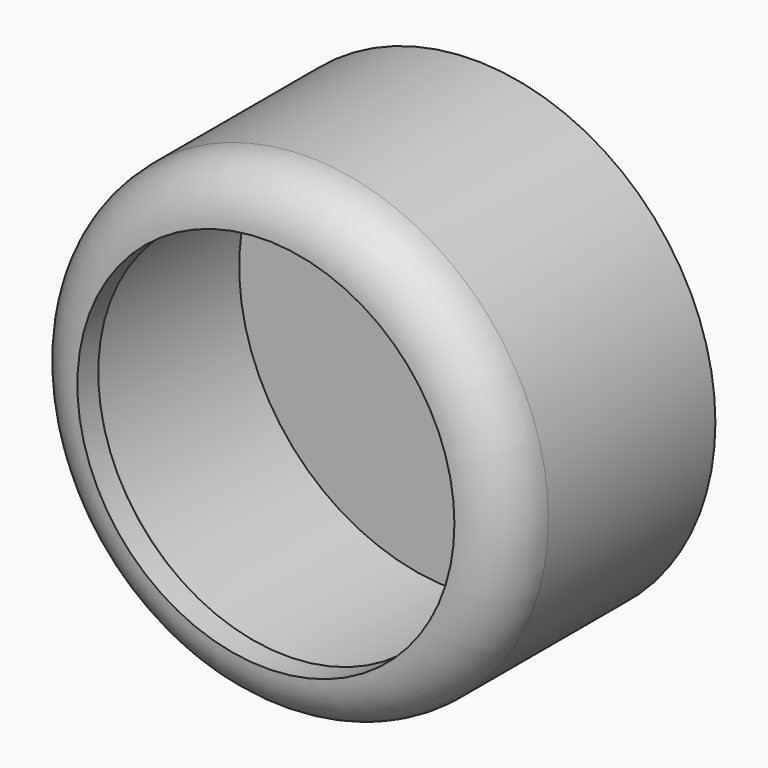
from build123d import *

# Parameters (mm, degrees)
F2_R     = 23.428989388
F3_DEPTH = 25.4
F4_R     = 5.08
F5_T     = -2.54


# Not quite as in the source:
# - a shell that OpenCascade refuses in one call is made with other operations: the cavity is built on its own and cut out
# - the program builds the solid bodies; features that only make, move or delete a surface that nothing else refers to are left out


with BuildPart() as f3:
    # F2 (on Front) → F3 (new body)
    with BuildSketch(Plane.XZ):
        with Locations((0, 28.4662228078)):
            Circle(F2_R)
    extrude(amount=F3_DEPTH)

    # F4
    f4_edges = [f3.edges().sort_by_distance(p)[0] for p in [
        (-23.428989, -25.4, 28.466223),
    ]]
    fillet(f4_edges, radius=F4_R)

    # F5: a shell. OpenCascade refuses it in one call, so the cavity is built on its own and cut out:
    # the body offset inwards by the wall thickness, plus a prism from it out through each open face.
    f5_core = offset(f3.part, amount=F5_T, mode=Mode.PRIVATE)
    f5_exits = [f5_core.faces().sort_by_distance(p)[0] for p in [
        (0, -22.86, 28.466223),
    ]]
    add(f5_core, mode=Mode.SUBTRACT)
    extrude(f5_exits, amount=-F5_T, mode=Mode.SUBTRACT)


solid = f3.part
